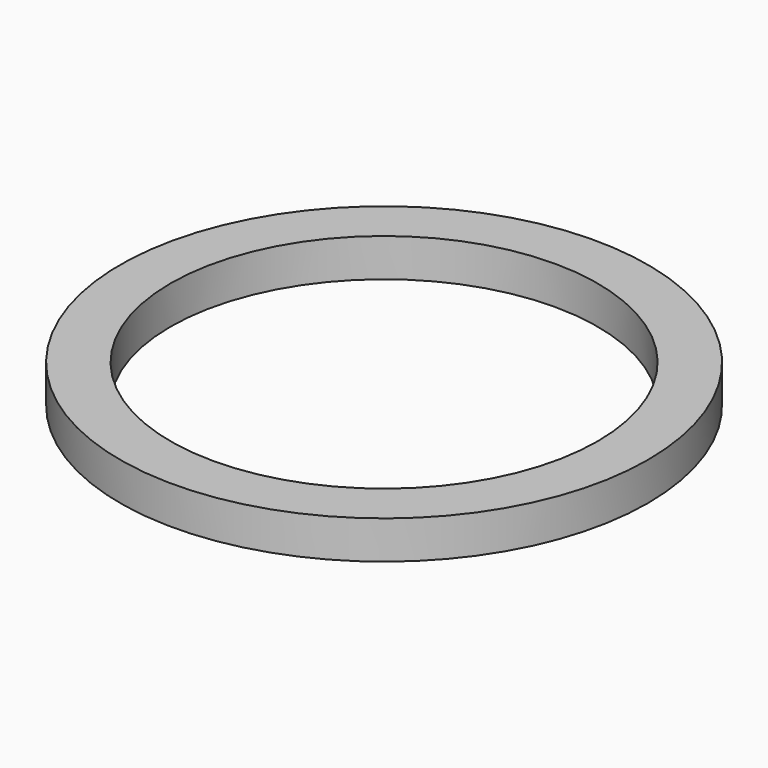
from build123d import *

# Parameters (mm, degrees)
F0_R     = 131.9530761388
F0_R_2   = 106.7955648348
F1_DEPTH = 19.05


# Not quite as in the source:
# - a feature names something its author has since deleted; it is built from what else it names


with BuildPart() as f1:
    # F0 (on Top) → F1 (new body)
    with BuildSketch(Plane.XY):
        Circle(F0_R)
        Circle(F0_R_2, mode=Mode.SUBTRACT)
    extrude(amount=F1_DEPTH)


solid = f1.part
